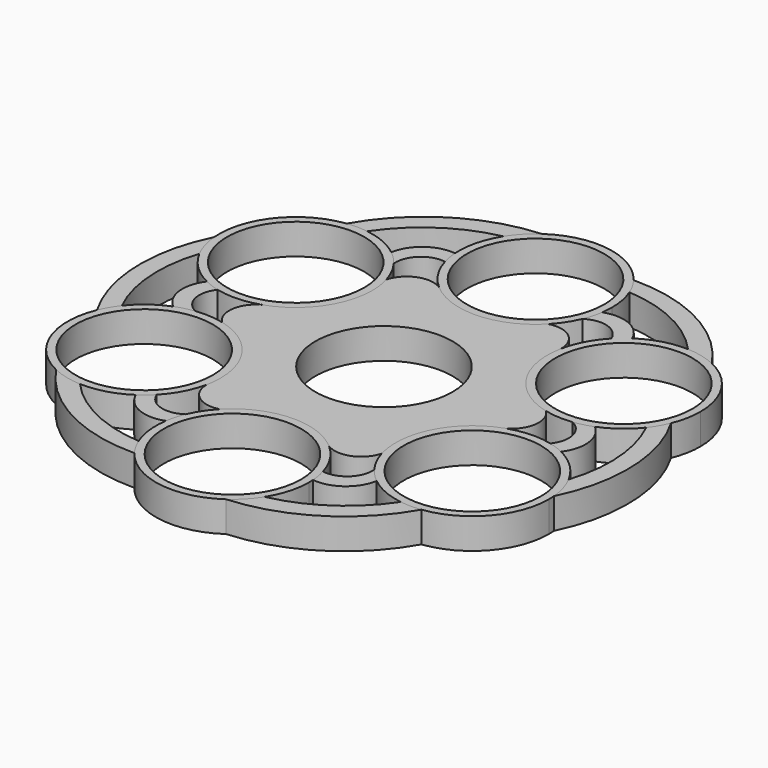
from build123d import *

# Parameters (mm, degrees)
F0_R     = 11.2
F1_DEPTH = 5
F2_DEPTH = 5
F3_DEPTH = 5


# Not quite as in the source:
# - a feature names something its author has since deleted; it is built from what else it names


with BuildPart() as f1:
    # F0 (on Top) → F1 (new body)
    with BuildSketch(Plane.XY):
        with BuildLine():
            ThreePointArc((14.5226124904, 17.9241838723), (12.8538052661, 21.4779922706), (9.0053139153, 22.2549002485))
            ThreePointArc((9.0053139153, 22.2549002485), (0.5155445548, 18.4324579571), (-8.2614923303, 21.5390432821))
            ThreePointArc((-8.2614923303, 21.5390432821), (-12.1735842956, 21.8707180311), (-14.7706520163, 18.9262807439))
            ThreePointArc((-14.7706520163, 18.9262807439), (-14.4033637941, 17.2098643735), (-14.2801243623, 15.4589223877))
            ThreePointArc((-14.2801243623, 15.4589223877), (-16.6263013318, 8.1685261114), (-22.7841048207, 3.6148594098))
            ThreePointArc((-22.7841048207, 3.6148594098), (-25.0273895617, 0.3927257605), (-23.7759659315, -3.3286195046))
            ThreePointArc((-23.7759659315, -3.3286195046), (-16.9347636083, -7.7580662961), (-14.277881684, -15.4628068204))
            ThreePointArc((-14.277881684, -15.4628068204), (-14.3392148559, -16.699563684), (-14.5226124904, -17.9241838723))
            ThreePointArc((-14.5226124904, -17.9241838723), (-12.8538052661, -21.4779922706), (-9.0053139153, -22.2549002485))
            ThreePointArc((-9.0053139153, -22.2549002485), (-0.5155445548, -18.4324579571), (8.2614923303, -21.5390432821))
            ThreePointArc((8.2614923303, -21.5390432821), (12.1735842956, -21.8707180311), (14.7706520163, -18.9262807439))
            ThreePointArc((14.7706520163, -18.9262807439), (15.7052045676, -9.6627036598), (22.7841048207, -3.6148594098))
            ThreePointArc((22.7841048207, -3.6148594098), (25.0273895617, -0.3927257605), (23.7759659315, 3.3286195046))
            ThreePointArc((23.7759659315, 3.3286195046), (16.2207491224, 8.7697542973), (14.5226124904, 17.9241838723))
        make_face()
        Circle(F0_R, mode=Mode.SUBTRACT)
    extrude(amount=F1_DEPTH)


with BuildPart() as f1b:
    # F0 (on Top) → F1, piece 2 (new body)
    with BuildSketch(Plane.XY):
        with BuildLine():
            ThreePointArc((-12.0176018207, 27.4748255718), (-12.3156109951, 28.7697625044), (-12.4744754724, 30.0890172961))
            ThreePointArc((-12.4744754724, 30.0890172961), (-16.6991448207, 28.9596321924), (-18.9903738552, 25.234902494))
            ThreePointArc((-18.9903738552, 25.234902494), (-17.8305847638, 24.1856480609), (-16.8108979569, 22.9997794265))
            ThreePointArc((-16.8108979569, 22.9997794265), (-15.5001412135, 26.4004187044), (-12.0176018207, 27.4748255718))
        make_face()
    extrude(amount=F1_DEPTH)


with BuildPart() as f1c:
    # F0 (on Top) → F1, piece 3 (new body)
    with BuildSketch(Plane.XY):
        with BuildLine():
            ThreePointArc((-10.577804923, 37.5856232053), (-9.042809868, 39.5541185001), (-7.1472808385, 41.1783577813))
            ThreePointArc((-7.1472808385, 41.1783577813), (-19.4516559982, 37.2034806966), (-28.3853619381, 27.8554223907))
            ThreePointArc((-28.3853619381, 27.8554223907), (-26.6938832134, 27.9586248827), (-25.0039895325, 27.8320927602))
            ThreePointArc((-25.0039895325, 27.8320927602), (-18.745164056, 34.1202883881), (-10.577804923, 37.5856232053))
        make_face()
    extrude(amount=F1_DEPTH)


with BuildPart() as f1d:
    # F0 (on Top) → F1, piece 4 (new body)
    with BuildSketch(Plane.XY):
        with BuildLine():
            ThreePointArc((9.9308224545, 38.5101557294), (10.8659377966, 37.0968934298), (11.6013046045, 35.5701365112))
            ThreePointArc((11.6013046045, 35.5701365112), (20.1764545006, 33.2939324646), (27.2612020514, 27.9534593823))
            ThreePointArc((27.2612020514, 27.9534593823), (29.7334665114, 27.6083623173), (32.0878635055, 26.7789056648))
            ThreePointArc((32.0878635055, 26.7789056648), (22.4933313933, 35.4473685884), (9.9308224545, 38.5101557294))
        make_face()
    extrude(amount=F1_DEPTH)


with BuildPart() as f1e:
    # F0 (on Top) → F1, piece 5 (new body)
    with BuildSketch(Plane.XY):
        with BuildLine():
            ThreePointArc((39.235144344, -14.3994521166), (41.9449873915, -1.7561121082), (38.3161843926, 10.6547333386))
            ThreePointArc((38.3161843926, 10.6547333386), (37.55982101, 9.1382685471), (36.6052941371, 7.738043751))
            ThreePointArc((36.6052941371, 7.738043751), (38.9216185566, -0.8263559235), (37.8390069744, -9.632163823))
            ThreePointArc((37.8390069744, -9.632163823), (38.7762763793, -11.9457561828), (39.235144344, -14.3994521166))
        make_face()
    extrude(amount=F1_DEPTH)


with BuildPart() as f1f:
    # F0 (on Top) → F1, piece 6 (new body)
    with BuildSketch(Plane.XY):
        with BuildLine():
            ThreePointArc((31.3492535494, 3.828694939), (29.8606780096, 3.3489153393), (28.3238422432, 3.0587749779))
            ThreePointArc((28.3238422432, 3.0587749779), (30.6135038753, 0.223306701), (29.8026978201, -3.3298643166))
            ThreePointArc((29.8026978201, -3.3298643166), (31.0731506872, -3.7192492673), (32.2950910896, -4.2412959901))
            ThreePointArc((32.2950910896, -4.2412959901), (33.4293495732, -0.01793246), (31.3492535494, 3.828694939))
        make_face()
    extrude(amount=F1_DEPTH)


with BuildPart() as f1g:
    # F0 (on Top) → F1, piece 7 (new body)
    with BuildSketch(Plane.XY):
        with BuildLine():
            ThreePointArc((7.1472808385, -41.1783577813), (19.4516559982, -37.2034806966), (28.3853619381, -27.8554223907))
            ThreePointArc((28.3853619381, -27.8554223907), (26.6938832134, -27.9586248827), (25.0039895325, -27.8320927602))
            ThreePointArc((25.0039895325, -27.8320927602), (18.745164056, -34.1202883881), (10.577804923, -37.5856232053))
            ThreePointArc((10.577804923, -37.5856232053), (9.042809868, -39.5541185001), (7.1472808385, -41.1783577813))
        make_face()
    extrude(amount=F1_DEPTH)


with BuildPart() as f1h:
    # F0 (on Top) → F1, piece 8 (new body)
    with BuildSketch(Plane.XY):
        with BuildLine():
            ThreePointArc((18.9903738552, -25.234902494), (17.8305847638, -24.1856480609), (16.8108979569, -22.9997794265))
            ThreePointArc((16.8108979569, -22.9997794265), (15.5001412135, -26.4004187044), (12.0176018207, -27.4748255718))
            ThreePointArc((12.0176018207, -27.4748255718), (12.3156109951, -28.7697625044), (12.4744754724, -30.0890172961))
            ThreePointArc((12.4744754724, -30.0890172961), (16.6991448207, -28.9596321924), (18.9903738552, -25.234902494))
        make_face()
    extrude(amount=F1_DEPTH)


with BuildPart() as f1i:
    # F0 (on Top) → F1, piece 9 (new body)
    with BuildSketch(Plane.XY):
        with BuildLine():
            ThreePointArc((-27.2612020514, -27.9534593823), (-29.7334665114, -27.6083623173), (-32.0878635055, -26.7789056648))
            ThreePointArc((-32.0878635055, -26.7789056648), (-22.4933313933, -35.4473685884), (-9.9308224545, -38.5101557294))
            ThreePointArc((-9.9308224545, -38.5101557294), (-10.8659377966, -37.0968934298), (-11.6013046045, -35.5701365112))
            ThreePointArc((-11.6013046045, -35.5701365112), (-20.1764545006, -33.2939324646), (-27.2612020514, -27.9534593823))
        make_face()
    extrude(amount=F1_DEPTH)


with BuildPart() as f1j:
    # F0 (on Top) → F1, piece 10 (new body)
    with BuildSketch(Plane.XY):
        with BuildLine():
            ThreePointArc((-17.7850959994, -24.1449612552), (-18.7575396921, -25.0505132371), (-19.8206156171, -25.8477213061))
            ThreePointArc((-19.8206156171, -25.8477213061), (-16.7302047525, -28.9416997324), (-12.3588796942, -29.063597433))
            ThreePointArc((-12.3588796942, -29.063597433), (-12.0300932458, -27.5345634002), (-11.5129442863, -26.0585544044))
            ThreePointArc((-11.5129442863, -26.0585544044), (-15.1133626618, -26.6237254054), (-17.7850959994, -24.1449612552))
        make_face()
    extrude(amount=F1_DEPTH)


with BuildPart() as f1k:
    # F0 (on Top) → F1, piece 11 (new body)
    with BuildSketch(Plane.XY):
        with BuildLine():
            ThreePointArc((-37.8390069744, 9.632163823), (-38.7762763793, 11.9457561828), (-39.235144344, 14.3994521166))
            ThreePointArc((-39.235144344, 14.3994521166), (-41.9449873915, 1.7561121082), (-38.3161843926, -10.6547333386))
            ThreePointArc((-38.3161843926, -10.6547333386), (-37.55982101, -9.1382685471), (-36.6052941371, -7.738043751))
            ThreePointArc((-36.6052941371, -7.738043751), (-38.9216185566, 0.8263559235), (-37.8390069744, 9.632163823))
        make_face()
    extrude(amount=F1_DEPTH)


with BuildPart() as f1l:
    # F0 (on Top) → F1, piece 12 (new body)
    with BuildSketch(Plane.XY):
        with BuildLine():
            ThreePointArc((-29.8026978201, 3.3298643166), (-31.0731506872, 3.7192492673), (-32.2950910896, 4.2412959901))
            ThreePointArc((-32.2950910896, 4.2412959901), (-33.4293495732, 0.01793246), (-31.3492535494, -3.828694939))
            ThreePointArc((-31.3492535494, -3.828694939), (-29.8606780096, -3.3489153393), (-28.3238422432, -3.0587749779))
            ThreePointArc((-28.3238422432, -3.0587749779), (-30.6135038753, -0.223306701), (-29.8026978201, 3.3298643166))
        make_face()
    extrude(amount=F1_DEPTH)


with BuildPart() as f2:
    # F0 (on Top) → F2 (new body)
    with BuildSketch(Plane.XY):
        with BuildLine():
            ThreePointArc((-25.0039895325, 27.8320927602), (-26.6938832134, 27.9586248827), (-28.3853619381, 27.8554223907))
            ThreePointArc((-28.3853619381, 27.8554223907), (-36.5109256988, 23.3050364163), (-39.235144344, 14.3994521166))
            ThreePointArc((-39.235144344, 14.3994521166), (-38.7762763793, 11.9457561828), (-37.8390069744, 9.632163823))
            ThreePointArc((-37.8390069744, 9.632163823), (-35.4943933781, 6.4972531503), (-32.2950910896, 4.2412959901))
            ThreePointArc((-32.2950910896, 4.2412959901), (-31.0731506872, 3.7192492673), (-29.8026978201, 3.3298643166))
            ThreePointArc((-29.8026978201, 3.3298643166), (-26.2729706673, 2.9692148199), (-22.7841048207, 3.6148594098))
            ThreePointArc((-22.7841048207, 3.6148594098), (-16.6263013318, 8.1685261114), (-14.2801243623, 15.4589223877))
            ThreePointArc((-14.2801243623, 15.4589223877), (-14.4033637941, 17.2098643735), (-14.7706520163, 18.9262807439))
            ThreePointArc((-14.7706520163, 18.9262807439), (-15.6036245712, 21.0567659386), (-16.8108979569, 22.9997794265))
            ThreePointArc((-16.8108979569, 22.9997794265), (-17.8305847638, 24.1856480609), (-18.9903738552, 25.234902494))
            ThreePointArc((-18.9903738552, 25.234902494), (-21.8240281274, 26.9344228174), (-25.0039895325, 27.8320927602))
        make_face()
        with Locations((-26.7801243623, 15.4589223877)):
            Circle(F0_R, mode=Mode.SUBTRACT)
    extrude(amount=F2_DEPTH)


with BuildPart() as f2b:
    # F0 (on Top) → F2, piece 2 (new body)
    with BuildSketch(Plane.XY):
        with BuildLine():
            ThreePointArc((32.0878635055, 26.7789056648), (29.7334665114, 27.6083623173), (27.2612020514, 27.9534593823))
            ThreePointArc((27.2612020514, 27.9534593823), (23.373982972, 27.4904197822), (19.8206156171, 25.8477213061))
            ThreePointArc((19.8206156171, 25.8477213061), (18.7575396921, 25.0505132371), (17.7850959994, 24.1449612552))
            ThreePointArc((17.7850959994, 24.1449612552), (15.707900797, 21.2684526209), (14.5226124904, 17.9241838723))
            ThreePointArc((14.5226124904, 17.9241838723), (16.2207491224, 8.7697542973), (23.7759659315, 3.3286195046))
            ThreePointArc((23.7759659315, 3.3286195046), (26.03750651, 2.9847523005), (28.3238422432, 3.0587749779))
            ThreePointArc((28.3238422432, 3.0587749779), (29.8606780096, 3.3489153393), (31.3492535494, 3.828694939))
            ThreePointArc((31.3492535494, 3.828694939), (34.2379084598, 5.4329513626), (36.6052941371, 7.738043751))
            ThreePointArc((36.6052941371, 7.738043751), (37.55982101, 9.1382685471), (38.3161843926, 10.6547333386))
            ThreePointArc((38.3161843926, 10.6547333386), (39.0350996362, 13.0111526703), (39.277881684, 15.4628068204))
            ThreePointArc((39.277881684, 15.4628068204), (37.3283502226, 22.1663591336), (32.0878635055, 26.7789056648))
        make_face()
        with Locations((26.777881684, 15.4628068204)):
            Circle(F0_R, mode=Mode.SUBTRACT)
        with BuildLine():
            ThreePointArc((19.8206156171, 25.8477213061), (16.7302047525, 28.9416997324), (12.3588796942, 29.063597433))
            ThreePointArc((12.3588796942, 29.063597433), (12.0300932458, 27.5345634002), (11.5129442863, 26.0585544044))
            ThreePointArc((11.5129442863, 26.0585544044), (15.1133626618, 26.6237254054), (17.7850959994, 24.1449612552))
            ThreePointArc((17.7850959994, 24.1449612552), (18.7575396921, 25.0505132371), (19.8206156171, 25.8477213061))
        make_face()
    extrude(amount=F2_DEPTH)


with BuildPart() as f2c:
    # F0 (on Top) → F2, piece 3 (new body)
    with BuildSketch(Plane.XY):
        with BuildLine():
            ThreePointArc((39.2801243623, -15.4589223877), (39.2688742951, -14.9287100582), (39.235144344, -14.3994521166))
            ThreePointArc((39.235144344, -14.3994521166), (38.7762763793, -11.9457561828), (37.8390069744, -9.632163823))
            ThreePointArc((37.8390069744, -9.632163823), (35.4943933781, -6.4972531503), (32.2950910896, -4.2412959901))
            ThreePointArc((32.2950910896, -4.2412959901), (31.0731506872, -3.7192492673), (29.8026978201, -3.3298643166))
            ThreePointArc((29.8026978201, -3.3298643166), (26.2729706673, -2.9692148199), (22.7841048207, -3.6148594098))
            ThreePointArc((22.7841048207, -3.6148594098), (15.7052045676, -9.6627036598), (14.7706520163, -18.9262807439))
            ThreePointArc((14.7706520163, -18.9262807439), (15.6036245712, -21.0567659386), (16.8108979569, -22.9997794265))
            ThreePointArc((16.8108979569, -22.9997794265), (17.8305847638, -24.1856480609), (18.9903738552, -25.234902494))
            ThreePointArc((18.9903738552, -25.234902494), (21.8240281274, -26.9344228174), (25.0039895325, -27.8320927602))
            ThreePointArc((25.0039895325, -27.8320927602), (26.6938832134, -27.9586248827), (28.3853619381, -27.8554223907))
            ThreePointArc((28.3853619381, -27.8554223907), (36.1693594136, -23.7107261391), (39.2801243623, -15.4589223877))
        make_face()
        with Locations((26.7801243623, -15.4589223877)):
            Circle(F0_R, mode=Mode.SUBTRACT)
    extrude(amount=F2_DEPTH)


with BuildPart() as f2d:
    # F0 (on Top) → F2, piece 4 (new body)
    with BuildSketch(Plane.XY):
        with BuildLine():
            ThreePointArc((-11.6013046045, -35.5701365112), (-10.8659377966, -37.0968934298), (-9.9308224545, -38.5101557294))
            ThreePointArc((-9.9308224545, -38.5101557294), (-1.9272907232, -43.271907379), (7.1472808385, -41.1783577813))
            ThreePointArc((7.1472808385, -41.1783577813), (9.042809868, -39.5541185001), (10.577804923, -37.5856232053))
            ThreePointArc((10.577804923, -37.5856232053), (12.0115001087, -34.3898318551), (12.5022426783, -30.9217292081))
            ThreePointArc((12.5022426783, -30.9217292081), (12.4952989482, -30.5051418385), (12.4744754724, -30.0890172961))
            ThreePointArc((12.4744754724, -30.0890172961), (12.3156109951, -28.7697625044), (12.0176018207, -27.4748255718))
            ThreePointArc((12.0176018207, -27.4748255718), (10.5650698704, -24.2376674407), (8.2614923303, -21.5390432821))
            ThreePointArc((8.2614923303, -21.5390432821), (-0.5155445548, -18.4324579571), (-9.0053139153, -22.2549002485))
            ThreePointArc((-9.0053139153, -22.2549002485), (-10.4338819388, -24.0415182391), (-11.5129442863, -26.0585544044))
            ThreePointArc((-11.5129442863, -26.0585544044), (-12.0300932458, -27.5345634002), (-12.3588796942, -29.063597433))
            ThreePointArc((-12.3588796942, -29.063597433), (-12.4138803324, -32.3673741799), (-11.6013046045, -35.5701365112))
        make_face()
        with Locations((0.0022426783, -30.9217292081)):
            Circle(F0_R, mode=Mode.SUBTRACT)
    extrude(amount=F2_DEPTH)


with BuildPart() as f2e:
    # F0 (on Top) → F2, piece 5 (new body)
    with BuildSketch(Plane.XY):
        with BuildLine():
            ThreePointArc((-36.6052941371, -7.738043751), (-37.55982101, -9.1382685471), (-38.3161843926, -10.6547333386))
            ThreePointArc((-38.3161843926, -10.6547333386), (-38.438216422, -19.9668709627), (-32.0878635055, -26.7789056648))
            ThreePointArc((-32.0878635055, -26.7789056648), (-29.7334665114, -27.6083623173), (-27.2612020514, -27.9534593823))
            ThreePointArc((-27.2612020514, -27.9534593823), (-23.373982972, -27.4904197822), (-19.8206156171, -25.8477213061))
            ThreePointArc((-19.8206156171, -25.8477213061), (-18.7575396921, -25.0505132371), (-17.7850959994, -24.1449612552))
            ThreePointArc((-17.7850959994, -24.1449612552), (-15.707900797, -21.2684526209), (-14.5226124904, -17.9241838723))
            ThreePointArc((-14.5226124904, -17.9241838723), (-14.3392148559, -16.699563684), (-14.277881684, -15.4628068204))
            ThreePointArc((-14.277881684, -15.4628068204), (-16.9347636083, -7.7580662961), (-23.7759659315, -3.3286195046))
            ThreePointArc((-23.7759659315, -3.3286195046), (-26.03750651, -2.9847523005), (-28.3238422432, -3.0587749779))
            ThreePointArc((-28.3238422432, -3.0587749779), (-29.8606780096, -3.3489153393), (-31.3492535494, -3.828694939))
            ThreePointArc((-31.3492535494, -3.828694939), (-34.2379084598, -5.4329513626), (-36.6052941371, -7.738043751))
        make_face()
        with Locations((-26.777881684, -15.4628068204)):
            Circle(F0_R, mode=Mode.SUBTRACT)
    extrude(amount=F2_DEPTH)


with BuildPart() as f3:
    # F0 (on Top) → F3 (new body)
    with BuildSketch(Plane.XY):
        with BuildLine():
            ThreePointArc((12.3588796942, 29.063597433), (12.462989563, 29.9900719899), (12.4977573217, 30.9217292081))
            ThreePointArc((12.4977573217, 30.9217292081), (12.271598225, 33.2887588831), (11.6013046045, 35.5701365112))
            ThreePointArc((11.6013046045, 35.5701365112), (10.8659377966, 37.0968934298), (9.9308224545, 38.5101557294))
            ThreePointArc((9.9308224545, 38.5101557294), (1.9272907232, 43.271907379), (-7.1472808385, 41.1783577813))
            ThreePointArc((-7.1472808385, 41.1783577813), (-9.042809868, 39.5541185001), (-10.577804923, 37.5856232053))
            ThreePointArc((-10.577804923, 37.5856232053), (-12.1204104061, 33.9876729325), (-12.4744754724, 30.0890172961))
            ThreePointArc((-12.4744754724, 30.0890172961), (-12.3156109951, 28.7697625044), (-12.0176018207, 27.4748255718))
            ThreePointArc((-12.0176018207, 27.4748255718), (-10.5650698704, 24.2376674407), (-8.2614923303, 21.5390432821))
            ThreePointArc((-8.2614923303, 21.5390432821), (0.5155445548, 18.4324579571), (9.0053139153, 22.2549002485))
            ThreePointArc((9.0053139153, 22.2549002485), (10.4338819388, 24.0415182391), (11.5129442863, 26.0585544044))
            ThreePointArc((11.5129442863, 26.0585544044), (12.0300932458, 27.5345634002), (12.3588796942, 29.063597433))
        make_face()
        with Locations((-0.0022426783, 30.9217292081)):
            Circle(F0_R, mode=Mode.SUBTRACT)
    extrude(amount=F3_DEPTH)


solid = Compound([f1.part, f1b.part, f1c.part, f1d.part, f1e.part, f1f.part, f1g.part, f1h.part, f1i.part, f1j.part, f1k.part, f1l.part, f2.part, f2b.part, f2c.part, f2d.part, f2e.part, f3.part])
